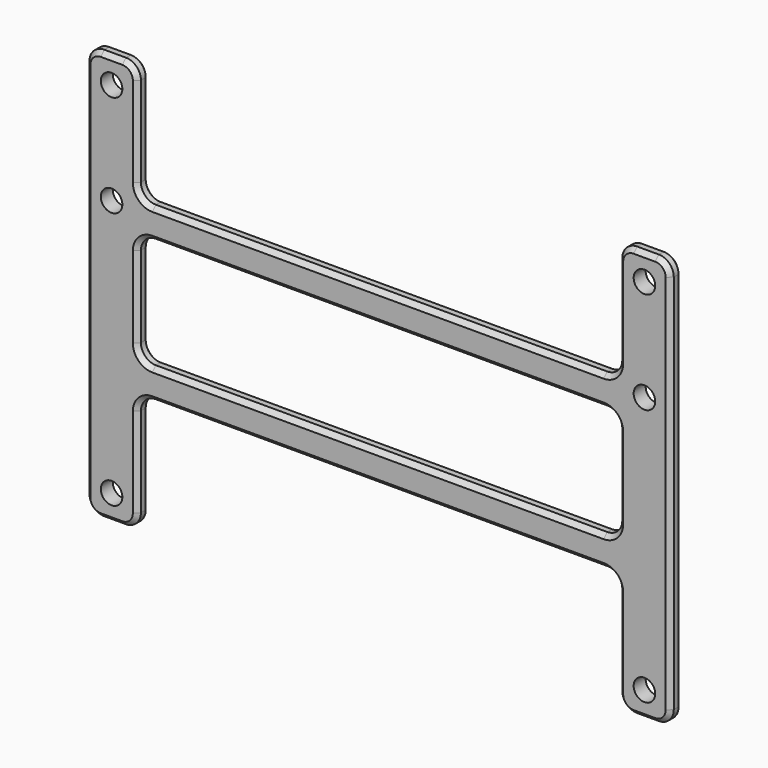
from build123d import *

# Parameters (mm, degrees)
F0_W     = 0.0285906434
F0_H     = 5
F0_W_2   = 40.2
F0_R     = 1.8
F1_DEPTH = 2.5
F2_R     = 2.5
F3_SIZE  = 0.75


# Not quite as in the source:
# - a feature names something its author has since deleted; it is built from what else it names


with BuildPart() as f1:
    # F0 (on Front) → F1 (new body)
    with BuildSketch(Plane.XZ):
        with Locations((-40.2142953217, 18.525)):
            Rectangle(F0_W, F0_H)
        with Locations((40.2142953217, 18.525)):
            Rectangle(F0_W, F0_H)
        with Locations((-20.1, 18.525)):
            Rectangle(F0_W_2, F0_H)
        with Locations((20.1, 18.525)):
            Rectangle(F0_W_2, F0_H)
        with Locations((20.1, 42.125)):
            Rectangle(F0_W_2, F0_H)
        Polygon((40.2, 64.625), (40.2, 44.625), (40.2, 39.625), (40.2, 21.025), (40.2285906434, 21.025), (40.2285906434, 16.025), (40.2, 16.025), (40.2, -3.975), (48.8, -3.975), (48.8, 64.625), align=None)
        with Locations((44.5, 0.325)):
            Circle(F0_R, mode=Mode.SUBTRACT)
        with Locations((44.5, 43.325)):
            Circle(F0_R, mode=Mode.SUBTRACT)
        with Locations((44.5, 60.325)):
            Circle(F0_R, mode=Mode.SUBTRACT)
        with Locations((-20.1, 42.125)):
            Rectangle(F0_W_2, F0_H)
        Polygon((-40.2, 64.625), (-48.8, 64.625), (-48.8, -3.975), (-40.2, -3.975), (-40.2, 16.025), (-40.2285906434, 16.025), (-40.2285906434, 21.025), (-40.2, 21.025), (-40.2, 39.625), (-40.2, 44.625), align=None)
        with Locations((-44.5, 0.325)):
            Circle(F0_R, mode=Mode.SUBTRACT)
        with Locations((-44.5, 43.325)):
            Circle(F0_R, mode=Mode.SUBTRACT)
        with Locations((-44.5, 60.325)):
            Circle(F0_R, mode=Mode.SUBTRACT)
    extrude(amount=F1_DEPTH)

    # F2
    f2_edges = [f1.edges().sort_by_distance(p)[0] for p in [
        (-40.2, -1.25, 44.625),
        (40.2, -1.25, 44.625),
        (-40.2, -1.25, 39.625),
        (40.2, -1.25, 39.625),
        (-40.2, -1.25, 21.025),
        (40.2, -1.25, 21.025),
        (-40.2, -1.25, 16.025),
        (40.2, -1.25, 16.025),
        (40.2, -1.25, -3.975),
        (48.8, -1.25, -3.975),
        (-48.8, -1.25, -3.975),
        (-40.2, -1.25, -3.975),
        (48.8, -1.25, 64.625),
        (40.2, -1.25, 64.625),
        (-48.8, -1.25, 64.625),
        (-40.2, -1.25, 64.625),
    ]]
    fillet(f2_edges, radius=F2_R)

    # F3
    f3_edges = [f1.edges().sort_by_distance(p)[0] for p in [
        (0, 0, 16.025),
        (0, 0, 39.625),
        (-44.5, -2.5, 64.625),
        (0, -2.5, 39.625),
    ]]
    chamfer(f3_edges, length=F3_SIZE)


solid = f1.part
